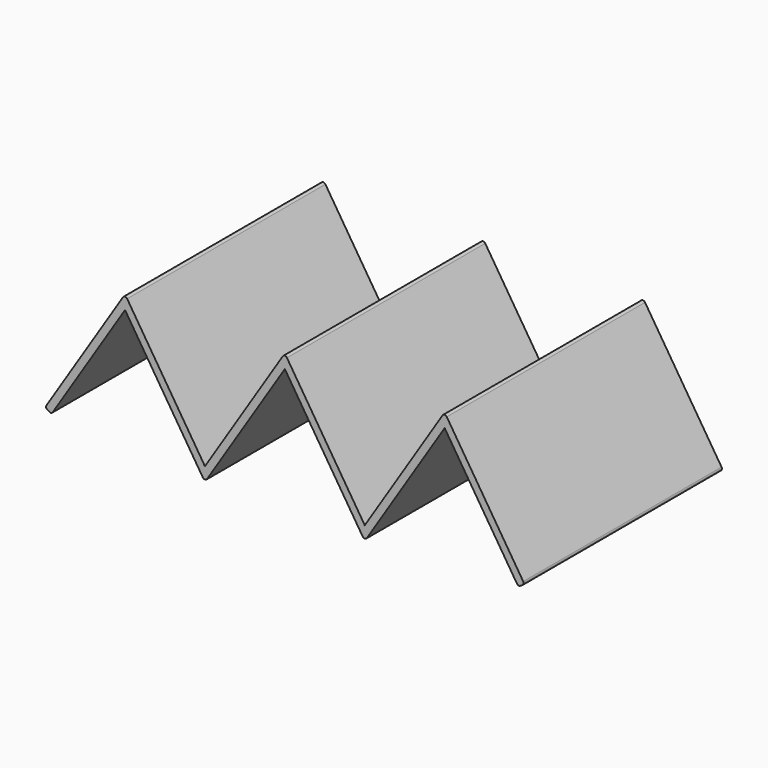
from build123d import *

# Parameters (mm, degrees)
F1_DEPTH = 100
F2_R     = 1


# Not quite as in the source:
# - ends of sketch curves that miss each other by under 0.0002 mm in the source are joined


with BuildPart() as f1:
    # F0 (on Front) → F1 (new body)
    with BuildSketch(Plane.XZ):
        Polygon((-75.7449854628, 50.6034867488), (-107.9829619636, 0), (-105.4527876261, -1.611898825), (-75.7449854628, 45.0200097587), (-43.5070133628, -5.5834700822), (-11.2690412628, 45.0200097587), (20.9689308372, -5.5834700822), (53.2069029372, 45.0200097587), (82.9147051006, -1.611898825), (85.444879438, 0), (53.2069029372, 50.6034867488), (20.9689264364, 0), (-11.2690412628, 50.6034867488), (-43.5070177636, 0), align=None)
    extrude(amount=F1_DEPTH)

    # F2
    f2_edges = [f1.edges().sort_by_distance(p)[0] for p in [
        (53.206903, -50, 50.603487),
        (-11.269041, -50, 50.603487),
        (-75.744985, -50, 50.603487),
        (-43.507013, -50, -5.58347),
        (20.968931, -50, -5.58347),
        (82.914705, -50, -1.611899),
        (-105.452788, -50, -1.611899),
        (-107.982962, -50, 0),
        (85.444879, -50, 0),
    ]]
    fillet(f2_edges, radius=F2_R)


solid = f1.part
